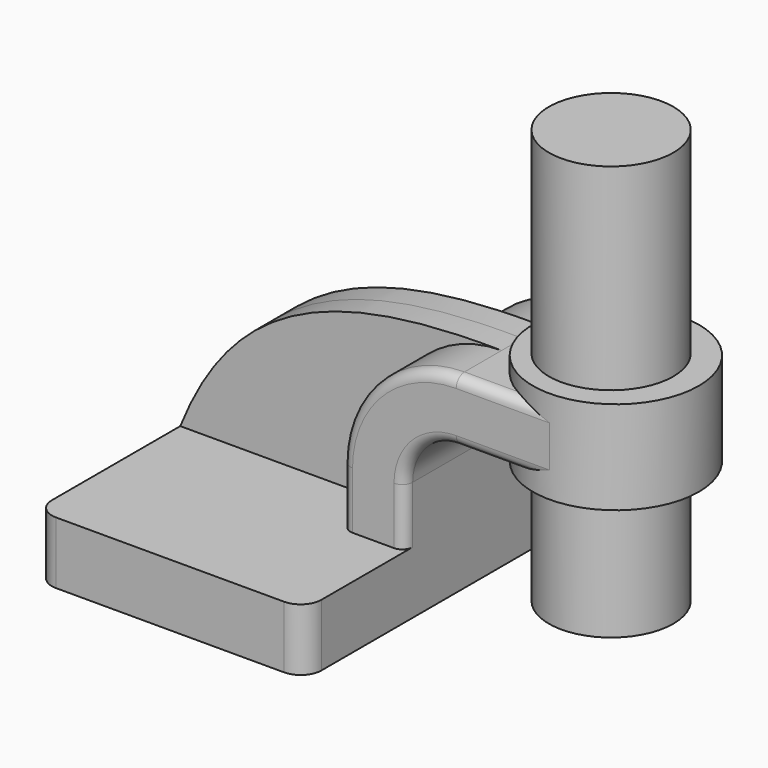
from build123d import *

# Parameters (mm, degrees)
F2_DEPTH     = 63.5
F0_W         = 25.4
F0_H         = 19.05
F3_DEPTH     = 25.4
F4_DEPTH     = 8.001
F6_R         = 6.35
F7_T1_DEPTH  = 17.4752
F7_T4_ANGLE  = 90
F7_T8_DEPTH  = 42.06875
F7_S9_R      = 25.4
F7_T10_DEPTH = 23
F7_T12_ANGLE = 90
F7_T14_ANGLE = 90
F7_T18_DEPTH = 42.06875
F7_S19_R     = 25.4
F7_T20_DEPTH = 23
F7_T22_ANGLE = 90
F7_T26_DEPTH = 42.06875
F7_S27_R     = 25.4
F7_T28_DEPTH = 23
F7_T32_DEPTH = 42.06875
F7_S33_R     = 25.4
F7_T34_DEPTH = 23
F8_R         = 19.05
F9_DEPTH     = 127


# Not quite as in the source:
# - a fillet or chamfer that OpenCascade refuses, or shapes differently, is made with other operations: its cross-section is extruded or revolved along the edge and cut away or added


with BuildPart() as f2:
    # F0 (on Front) → F2 (new body, symmetric)
    with BuildSketch(Plane.XZ):
        Polygon((22.225, 9.525), (-41.275, 9.525), (-41.275, -9.525), (41.275, -9.525), (41.275, 9.525), align=None)
    extrude(amount=F2_DEPTH, both=True)

    # F0 (on Front) → F3 (join, symmetric)
    with BuildSketch(Plane.XZ):
        with BuildLine():
            Line((22.225, 27.0002), (22.225, 9.525))
            Line((22.225, 9.525), (41.275, 9.525))
            Line((41.275, 9.525), (41.275, 27.0002))
            ThreePointArc((41.275, 27.0002), (45.9246798487, 38.2255201513), (57.15, 42.8752))
            Line((57.15, 42.8752), (60.325, 42.8752))
            Line((60.325, 42.8752), (60.325, 61.9252))
            Line((60.325, 61.9252), (57.15, 61.9252))
            ThreePointArc((57.15, 61.9252), (32.4542956671, 51.6959043329), (22.225, 27.0002))
        make_face()
        with Locations((73.025, 52.4002)):
            Rectangle(F0_W, F0_H)
    extrude(amount=F3_DEPTH, both=True)

    # F0 (on Front) → F4 (join, symmetric)
    with BuildSketch(Plane.XZ):
        with BuildLine():
            add(Edge.make_bspline(
                [(-41.275, 9.525), (-25.3429859877, 49.4523830712), (4.4616423547, 62.58662045), (57.15, 61.9252)],
                knots=[0, 0, 0, 0, 111.5045361635, 111.5045361635, 111.5045361635, 111.5045361635], degree=3))
            Line((-41.275, 9.525), (22.225, 9.525))
            Line((22.225, 9.525), (22.225, 27.0002))
            ThreePointArc((22.225, 27.0002), (32.4542956671, 51.6959043329), (57.15, 61.9252))
        make_face()
    extrude(amount=F4_DEPTH, both=True)

    # F0 (on Front) → F5 (revolve)
    with BuildSketch(Plane.XZ):
        Polygon((85.725, 66.675), (85.725, 61.9252), (85.725, 42.8752), (85.725, 38.1), (111.125, 38.1), (111.125, 66.675), align=None)
    revolve(axis=Axis((85.725, 0, 52.3875), (0, 0, 1)))

    # F6
    f6_edges = [f2.edges().sort_by_distance(p)[0] for p in [
        (41.275, -63.5, 0),
        (-41.275, -63.5, 0),
        (41.275, 63.5, 0),
        (-41.275, 63.5, 0),
    ]]
    fillet(f6_edges, radius=F6_R)

    # F7: fillet of radius 3.175 on 12 edges, made by hand

    # F7_s2 → F7_t1 (cut)
    with BuildSketch(Plane.XY.offset(9.525)):
        with BuildLine():
            ThreePointArc((25.4, -25.4), (23.1549359697, -24.4700640303), (22.225, -22.225))
            Line((22.225, -22.225), (22.225, -25.4))
            Line((22.225, -25.4), (25.4, -25.4))
        make_face()
        with BuildLine():
            ThreePointArc((41.275, -22.225), (40.3450640303, -24.4700640303), (38.1, -25.4))
            Line((38.1, -25.4), (41.275, -25.4))
            Line((41.275, -25.4), (41.275, -22.225))
        make_face()
        with BuildLine():
            ThreePointArc((25.4, 25.4), (23.1549359697, 24.4700640303), (22.225, 22.225))
            Line((22.225, 22.225), (22.225, 25.4))
            Line((22.225, 25.4), (25.4, 25.4))
        make_face()
        with BuildLine():
            ThreePointArc((41.275, 22.225), (40.3450640303, 24.4700640303), (38.1, 25.4))
            Line((38.1, 25.4), (41.275, 25.4))
            Line((41.275, 25.4), (41.275, 22.225))
        make_face()
    extrude(amount=F7_T1_DEPTH, mode=Mode.SUBTRACT)

    # F7_s3 → F7_t4 (revolve, cut)
    with BuildSketch(Plane.YZ.offset(57.15)):
        with BuildLine():
            ThreePointArc((-25.4, 58.7502), (-24.4700640303, 60.9952640303), (-22.225, 61.9252))
            Line((-22.225, 61.9252), (-25.4, 61.9252))
            Line((-25.4, 61.9252), (-25.4, 58.7502))
        make_face()
    revolve(axis=Axis((57.15, -25.4, 27.0002), (0, -1, 0)), revolution_arc=F7_T4_ANGLE, mode=Mode.SUBTRACT)


with BuildPart() as f7_tool6:
    # F7_s7 → F7_t8 (new body)
    with BuildSketch(Plane.YZ.offset(99.21875)):
        with BuildLine():
            ThreePointArc((-25.4, 58.7502), (-24.4700640303, 60.9952640303), (-22.225, 61.9252))
            Line((-22.225, 61.9252), (-25.4, 61.9252))
            Line((-25.4, 61.9252), (-25.4, 58.7502))
        make_face()
    extrude(amount=-F7_T8_DEPTH)

    # F7_s9 → F7_t10 (cut, symmetric)
    with BuildSketch(Plane.XY.offset(60.3)):
        with Locations((85.725, 0)):
            Circle(F7_S9_R)
    extrude(amount=F7_T10_DEPTH, both=True, mode=Mode.SUBTRACT)


with BuildPart() as f2_1:
    add(f2.part)

    # F7_t5: cut F7_tool6
    add(f7_tool6.part, mode=Mode.SUBTRACT)

    # F7_s11 → F7_t12 (revolve, cut)
    with BuildSketch(Plane.XY.offset(27.0002)):
        with BuildLine():
            ThreePointArc((41.275, -22.225), (40.3450640303, -24.4700640303), (38.1, -25.4))
            Line((38.1, -25.4), (41.275, -25.4))
            Line((41.275, -25.4), (41.275, -22.225))
        make_face()
    revolve(axis=Axis((57.15, -25.4, 27.0002), (0, 1, 0)), revolution_arc=F7_T12_ANGLE, mode=Mode.SUBTRACT)

    # F7_s13 → F7_t14 (revolve, cut)
    with BuildSketch(Plane.YZ.offset(57.15)):
        with BuildLine():
            ThreePointArc((25.4, 58.7502), (24.4700640303, 60.9952640303), (22.225, 61.9252))
            Line((22.225, 61.9252), (25.4, 61.9252))
            Line((25.4, 61.9252), (25.4, 58.7502))
        make_face()
    revolve(axis=Axis((57.15, 25.4, 27.0002), (0, -1, 0)), revolution_arc=F7_T14_ANGLE, mode=Mode.SUBTRACT)


with BuildPart() as f7_tool16:
    # F7_s17 → F7_t18 (new body)
    with BuildSketch(Plane.YZ.offset(99.21875)):
        with BuildLine():
            ThreePointArc((25.4, 58.7502), (24.4700640303, 60.9952640303), (22.225, 61.9252))
            Line((22.225, 61.9252), (25.4, 61.9252))
            Line((25.4, 61.9252), (25.4, 58.7502))
        make_face()
    extrude(amount=-F7_T18_DEPTH)

    # F7_s19 → F7_t20 (cut, symmetric)
    with BuildSketch(Plane.XY.offset(60.3)):
        with Locations((85.725, 0)):
            Circle(F7_S19_R)
    extrude(amount=F7_T20_DEPTH, both=True, mode=Mode.SUBTRACT)


with BuildPart() as f2_2:
    add(f2_1.part)

    # F7_t15: cut F7_tool16
    add(f7_tool16.part, mode=Mode.SUBTRACT)

    # F7_s21 → F7_t22 (revolve, cut)
    with BuildSketch(Plane.XY.offset(27.0002)):
        with BuildLine():
            ThreePointArc((38.1, 25.4), (40.3450640303, 24.4700640303), (41.275, 22.225))
            Line((41.275, 22.225), (41.275, 25.4))
            Line((41.275, 25.4), (38.1, 25.4))
        make_face()
    revolve(axis=Axis((57.15, 25.4, 27.0002), (0, 1, 0)), revolution_arc=F7_T22_ANGLE, mode=Mode.SUBTRACT)


with BuildPart() as f7_tool24:
    # F7_s25 → F7_t26 (new body)
    with BuildSketch(Plane.YZ.offset(57.15)):
        with BuildLine():
            ThreePointArc((25.4, 46.0502), (24.4700640303, 43.8051359697), (22.225, 42.8752))
            Line((22.225, 42.8752), (25.4, 42.8752))
            Line((25.4, 42.8752), (25.4, 46.0502))
        make_face()
    extrude(amount=F7_T26_DEPTH)

    # F7_s27 → F7_t28 (cut, symmetric)
    with BuildSketch(Plane.XY.offset(44.5)):
        with Locations((85.725, 0)):
            Circle(F7_S27_R)
    extrude(amount=F7_T28_DEPTH, both=True, mode=Mode.SUBTRACT)


with BuildPart() as f2_3:
    add(f2_2.part)

    # F7_t23: cut F7_tool24
    add(f7_tool24.part, mode=Mode.SUBTRACT)


with BuildPart() as f7_tool30:
    # F7_s31 → F7_t32 (new body)
    with BuildSketch(Plane.YZ.offset(57.15)):
        with BuildLine():
            ThreePointArc((-25.4, 46.0502), (-24.4700640303, 43.8051359697), (-22.225, 42.8752))
            Line((-22.225, 42.8752), (-25.4, 42.8752))
            Line((-25.4, 42.8752), (-25.4, 46.0502))
        make_face()
    extrude(amount=F7_T32_DEPTH)

    # F7_s33 → F7_t34 (cut, symmetric)
    with BuildSketch(Plane.XY.offset(44.5)):
        with Locations((85.725, 0)):
            Circle(F7_S33_R)
    extrude(amount=F7_T34_DEPTH, both=True, mode=Mode.SUBTRACT)


with BuildPart() as f2_4:
    add(f2_3.part)

    # F7_t29: cut F7_tool30
    add(f7_tool30.part, mode=Mode.SUBTRACT)

    # F8 (on Top) → F9 (join)
    with BuildSketch(Plane.XY):
        with Locations((84.2625681776, 0)):
            Circle(F8_R)
    extrude(amount=F9_DEPTH)


solid = f2_4.part
